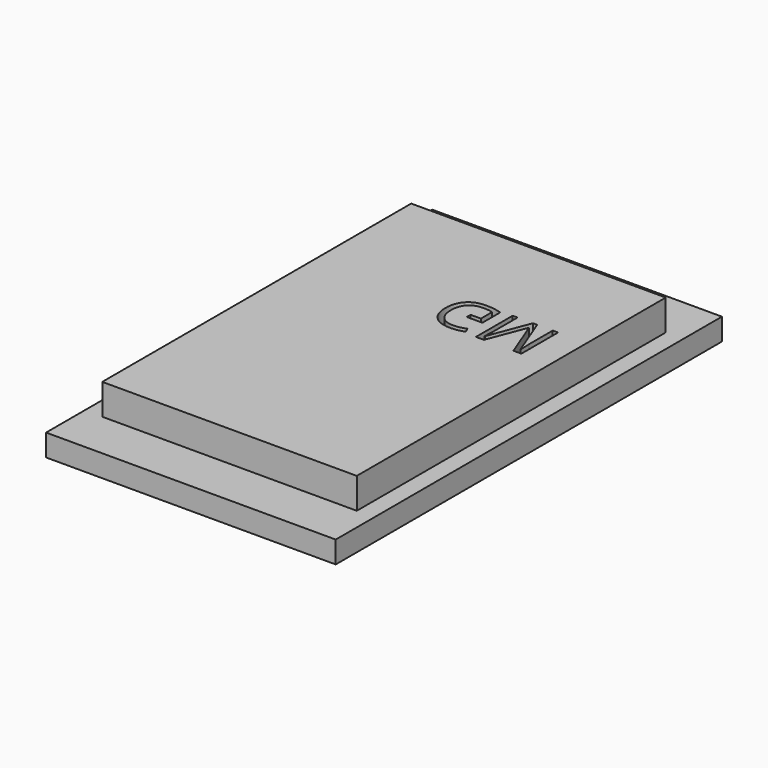
from build123d import *

# Parameters (mm, degrees)
F0_W         = 66
F0_H         = 110
F1_DEPTH     = 5
F2_W         = 58
F2_H         = 88
F3_DEPTH     = 7
F4_TEXT_SIZE = 14.6443300197
F5_DEPTH     = 38.7


# Not quite as in the source:
# - Text() gives the source's letters only with a copy of the font that has no kerning and outlines rounded to 1/6400 em; it was checked with that copy


with BuildPart() as f1:
    # F0 (on Top) → F1 (new body)
    with BuildSketch(Plane.XY):
        Rectangle(F0_W, F0_H)
    extrude(amount=F1_DEPTH)

    # F2 (on face) → F3 (join)
    with BuildSketch(Plane.XY.offset(5)):
        Rectangle(F2_W, F2_H)
    extrude(amount=F3_DEPTH)

    # F4 (on face) → F5 (cut)
    with BuildSketch(Plane(origin=(0, 0, 0), x_dir=(1, 0, 0), z_dir=(0, 0, -1))):
        with Locations((0, -21.5161352709)):
            Text('GM', F4_TEXT_SIZE, font='Open Sans', text_align=(TextAlign.LEFT, TextAlign.BOTTOM))
    extrude(amount=-F5_DEPTH, mode=Mode.SUBTRACT)


solid = f1.part
